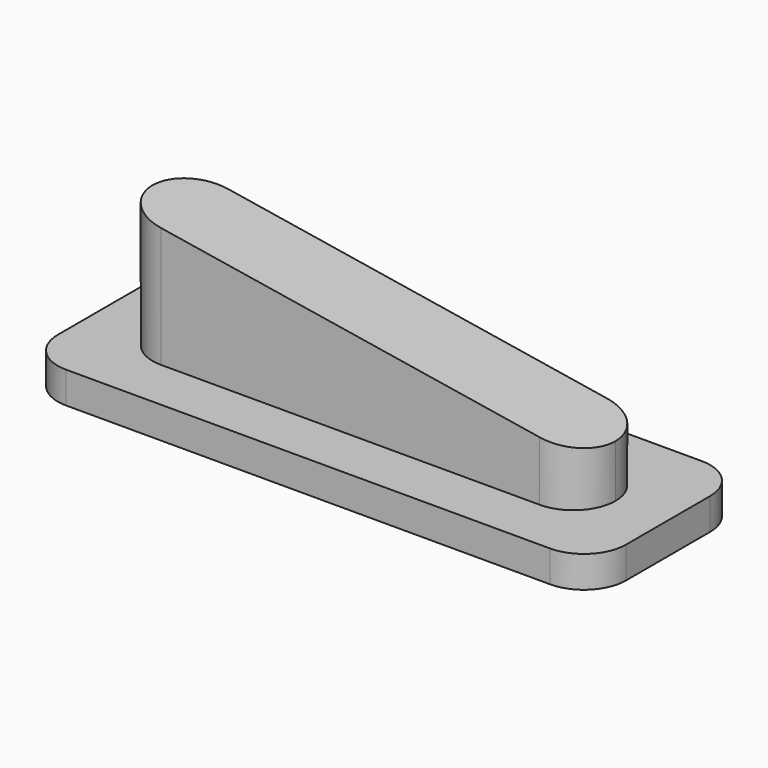
from build123d import *

# Parameters (mm, degrees)
F1_DEPTH = 4
F2_W     = 54
F2_H     = 18
F3_DEPTH = 3
F4_R     = 3.99999


# Not quite as in the source:
# - a fillet or chamfer is up to 0.001 mm smaller than in the source, because OpenCascade refuses the exact size


with BuildPart() as f1:
    # F0 (on Front) → F1 (new body, symmetric)
    with BuildSketch(Plane.XZ):
        Polygon((-49, 0), (5, 0), (5, 3), (0, 3), (0, 8), (-44, 15.1), (-44, 3), (-49, 3), align=None)
    extrude(amount=F1_DEPTH, both=True)

    # F2 (on face) → F3 (join, through all)
    with BuildSketch(Plane(origin=(0, 0, 0), x_dir=(1, 0, 0), z_dir=(0, 0, -1))):
        with Locations((-22, 0)):
            Rectangle(F2_W, F2_H)
    extrude(amount=-F3_DEPTH)

    # F4 (radius 4 in the source; OpenCascade refuses exactly that, so slightly less here)
    f4_edges = [f1.edges().sort_by_distance(p)[0] for p in [
        (0, -4, 5.5),
        (0, 4, 5.5),
        (-44, 4, 9.05),
        (-44, -4, 9.05),
        (-49, -9, 1.5),
        (-49, 9, 1.5),
        (5, 9, 1.5),
        (5, -9, 1.5),
    ]]
    fillet(f4_edges, radius=F4_R)


solid = f1.part
